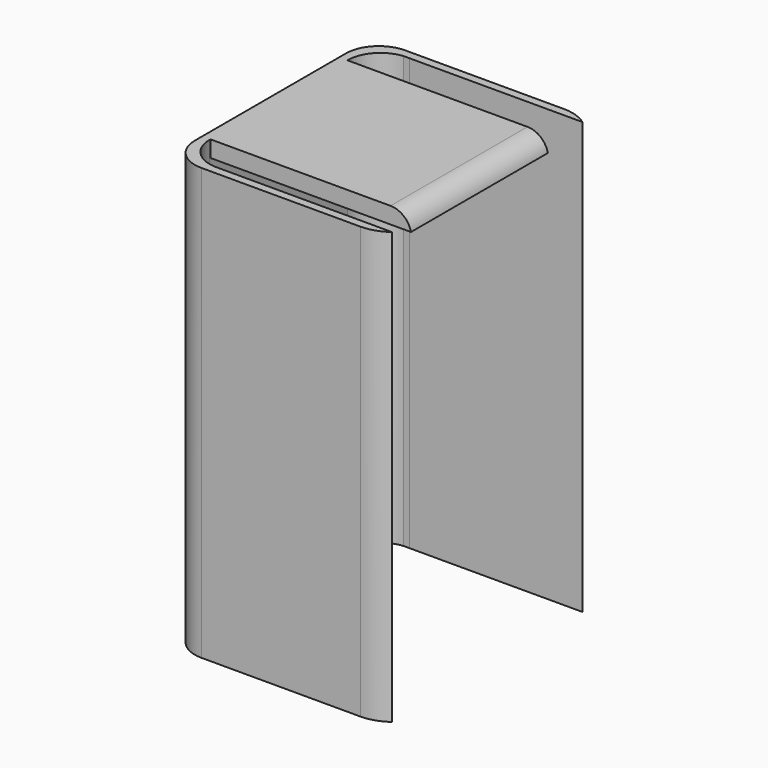
from build123d import *

# Parameters (mm, degrees)
F1_DEPTH    = 2
F2_DEPTH    = 103
F3_W        = 50.8
F3_H        = 41.6650772095
F4_DEPTH    = 2
F5_T1_DEPTH = 135.3099275981
F5_T3_DEPTH = 135.2654919008
F6_T1_DEPTH = 41.6650772095


# Not quite as in the source:
# - a fillet or chamfer that OpenCascade refuses, or shapes differently, is made with other operations: its cross-section is extruded or revolved along the edge and cut away or added
# - a feature names something its author has since deleted; it is built from what else it names


with BuildPart() as f1:
    # F0 (on Top) → F1 (new body)
    with BuildSketch(Plane.XY):
        with BuildLine():
            Line((23.2482, -29.5159982), (-19.5, -29.5159982))
            ThreePointArc((-19.5, -29.5159982), (-25.1568542495, -27.1728524495), (-27.5, -21.5159982))
            Line((-27.5, -21.5159982), (-27.5, 20.4840018))
            ThreePointArc((-27.5, 20.4840018), (-25.4213975047, 25.863318819), (-20.2657371023, 28.4472703934))
            Line((-20.2657371023, 28.4472703934), (-18.7638364732, 28.4472703934))
            Line((-18.7638364732, 28.4472703934), (23.2477635268, 28.4774018))
            Line((23.2477635268, 28.4774018), (23.2477635268, 30.4840018))
            Line((23.2477635268, 30.4840018), (-13.8766431592, 30.4840018))
            Line((-13.8766431592, 30.4840018), (-18.7638364732, 30.4840018))
            Line((-18.7638364732, 30.4840018), (-21.4966431592, 30.4840018))
            ThreePointArc((-21.4966431592, 30.4840018), (-27.1487639749, 28.1455855258), (-29.4966319659, 22.4973843711))
            Line((-29.4966319659, 22.4973843711), (-29.5, 20.4840018))
            Line((-29.5, 20.4840018), (-29.5, -21.5159982))
            Line((-29.5, -21.5159982), (-29.5, -23.5159982))
            ThreePointArc((-29.5, -23.5159982), (-27.1568542495, -29.1728524495), (-21.5, -31.5159982))
            Line((-21.5, -31.5159982), (-19.5, -31.5159982))
            Line((-19.5, -31.5159982), (23.2482, -31.5159982))
            Line((23.2482, -31.5159982), (23.2482, -29.5159982))
        make_face()
    extrude(amount=F1_DEPTH)

    # F0 (on Top) → F2 (join)
    with BuildSketch(Plane.XY):
        with BuildLine():
            Line((23.2482, -29.5159982), (-19.5, -29.5159982))
            ThreePointArc((-19.5, -29.5159982), (-25.1568542495, -27.1728524495), (-27.5, -21.5159982))
            Line((-27.5, -21.5159982), (-27.5, 20.4840018))
            ThreePointArc((-27.5, 20.4840018), (-25.4213975047, 25.863318819), (-20.2657371023, 28.4472703934))
            Line((-20.2657371023, 28.4472703934), (-18.7638364732, 28.4472703934))
            Line((-18.7638364732, 28.4472703934), (23.2477635268, 28.4774018))
            Line((23.2477635268, 28.4774018), (23.2477635268, 30.4840018))
            Line((23.2477635268, 30.4840018), (-13.8766431592, 30.4840018))
            Line((-13.8766431592, 30.4840018), (-18.7638364732, 30.4840018))
            Line((-18.7638364732, 30.4840018), (-21.4966431592, 30.4840018))
            ThreePointArc((-21.4966431592, 30.4840018), (-27.1487639749, 28.1455855258), (-29.4966319659, 22.4973843711))
            Line((-29.4966319659, 22.4973843711), (-29.5, 20.4840018))
            Line((-29.5, 20.4840018), (-29.5, -21.5159982))
            Line((-29.5, -21.5159982), (-29.5, -23.5159982))
            ThreePointArc((-29.5, -23.5159982), (-27.1568542495, -29.1728524495), (-21.5, -31.5159982))
            Line((-21.5, -31.5159982), (-19.5, -31.5159982))
            Line((-19.5, -31.5159982), (23.2482, -31.5159982))
            Line((23.2482, -31.5159982), (23.2482, -29.5159982))
        make_face()
    extrude(amount=-F2_DEPTH)

    # F3 (on Top) → F4 (join, symmetric)
    with BuildSketch(Plane.XY):
        with Locations((-4.1, -0.4146657884)):
            Rectangle(F3_W, F3_H)
    extrude(amount=F4_DEPTH, both=True)

    # F5: fillet of radius 10.16 on 2 edges, made by hand

    # F5_s2 → F5_t1 (cut)
    with BuildSketch(Plane.XY.offset(-118.154963799)):
        with BuildLine():
            ThreePointArc((17.1857780072, 30.4840018), (20.3785085, 29.9693152734), (23.2477635268, 28.4774018))
            Line((23.2477635268, 28.4774018), (23.2477635268, 30.4840018))
            Line((23.2477635268, 30.4840018), (17.1857780072, 30.4840018))
        make_face()
    extrude(amount=F5_T1_DEPTH, mode=Mode.SUBTRACT)

    # F5_s4 → F5_t3 (cut)
    with BuildSketch(Plane.XY.offset(-118.1327459504)):
        with BuildLine():
            ThreePointArc((17.1951016198, -31.5159982), (20.3825771099, -31.003049563), (23.2482, -29.5159982))
            Line((23.2482, -29.5159982), (23.2482, -31.5159982))
            Line((23.2482, -31.5159982), (17.1951016198, -31.5159982))
        make_face()
    extrude(amount=F5_T3_DEPTH, mode=Mode.SUBTRACT)

    # F6: fillet of radius 5.08 on 1 edges, made by hand

    # F6_s2 → F6_t1 (cut)
    with BuildSketch(Plane.XZ.offset(-20.4178728163)):
        with BuildLine():
            ThreePointArc((16.3361305416, 2), (19.5236060317, 0.8755530587), (21.3, -2))
            Line((21.3, -2), (21.3, 2))
            Line((21.3, 2), (16.3361305416, 2))
        make_face()
    extrude(amount=F6_T1_DEPTH, mode=Mode.SUBTRACT)


solid = f1.part
